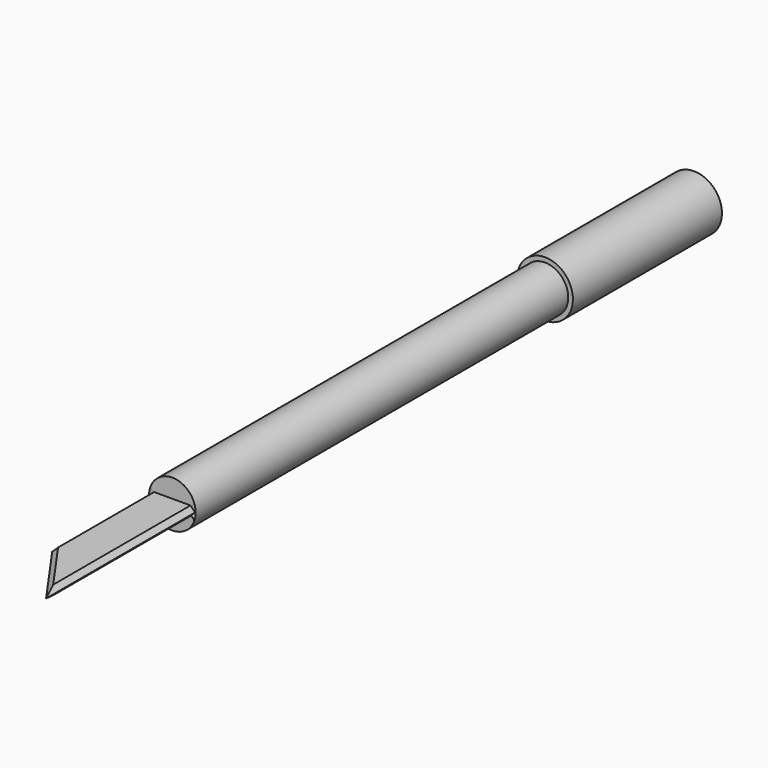
from build123d import *

# Parameters (mm, degrees)
F0_R       = 3.175
F1_DEPTH   = 88.9
F3_DEPTH   = 25.4
F5_DEPTH   = 25.4
F6_C1_SIZE = 0.635
F6_C2_SIZE = 0.635
F6_C3_SIZE = 0.635
F7_SIZE    = 0.63499
F8_DEPTH   = 25.4
F9_R       = 3.81
F9_R_2     = 3.175
F10_DEPTH  = 25.4


# Not quite as in the source:
# - a fillet or chamfer is up to 0.001 mm smaller than in the source, because OpenCascade refuses the exact size


with BuildPart() as f1:
    # F0 (on Front) → F1 (new body)
    with BuildSketch(Plane.XZ):
        Circle(F0_R)
    extrude(amount=F1_DEPTH)

    # F2 (on face) → F3 (join)
    with BuildSketch(Plane.XZ.offset(88.9)):
        Polygon((-1.5875, -0.635), (0, -0.635), (0, 0), (0, 0.635), (-1.5875, 0.635), (-3.1108519733, 0.635), (-3.1108519733, -0.635), align=None)
        Polygon((0, 0), (0, -0.635), (3.1108519733, -0.635), (3.1108519733, 0.635), (0, 0.635), align=None)
    extrude(amount=F3_DEPTH)

    # F4 (on face) → F5 (cut)
    with BuildSketch(Plane.XY.offset(0.635)):
        Polygon((-3.1108519733, -114.3), (3.1108519733, -114.3), (-3.1108519733, -105.4782980667), align=None)
    extrude(amount=-F5_DEPTH, mode=Mode.SUBTRACT)

    # F6: chamfer of 0.635 on 3 edges, made by hand

    # F6_c1
    f6_c1_edges = [f1.edges().sort_by_distance(p)[0] for p in [
        (3.1108519733, -101.6, 0.635),
    ]]
    chamfer(f6_c1_edges, length=F6_C1_SIZE)

    # F6_c2
    f6_c2_edges = [f1.edges().sort_by_distance(p)[0] for p in [
        (-3.1108519733, -97.1891490333, 0.635),
    ]]
    chamfer(f6_c2_edges, length=F6_C2_SIZE)

    # F6_c3
    f6_c3_edges = [f1.edges().sort_by_distance(p)[0] for p in [
        (0, -109.8891490333, 0.635),
    ]]
    chamfer(f6_c3_edges, length=F6_C3_SIZE)

    # F7 (size 0.635 in the source; OpenCascade refuses exactly that, so slightly less here)
    f7_edges = [f1.edges().sort_by_distance(p)[0] for p in [
        (0, -109.889149, -0.635),
        (-3.110852, -97.189149, -0.635),
        (3.110852, -101.6, -0.635),
    ]]
    chamfer(f7_edges, length=F7_SIZE)

    # F8 (cut): a face of the model
    f8_faces = [f1.faces().sort_by_distance(p)[0] for p in [
        (0, 0, 0),
    ]]
    extrude(f8_faces, amount=-F8_DEPTH, mode=Mode.SUBTRACT)


with BuildPart() as f10:
    # F9 (on face) → F10 (new body)
    with BuildSketch(Plane(origin=(0, -25.4, 0), x_dir=(-1, 0, 0), z_dir=(0, 1, 0))):
        Circle(F9_R)
        Circle(F9_R_2, mode=Mode.SUBTRACT)
        Circle(F9_R_2)
    extrude(amount=F10_DEPTH)


solid = Compound([f1.part, f10.part])
